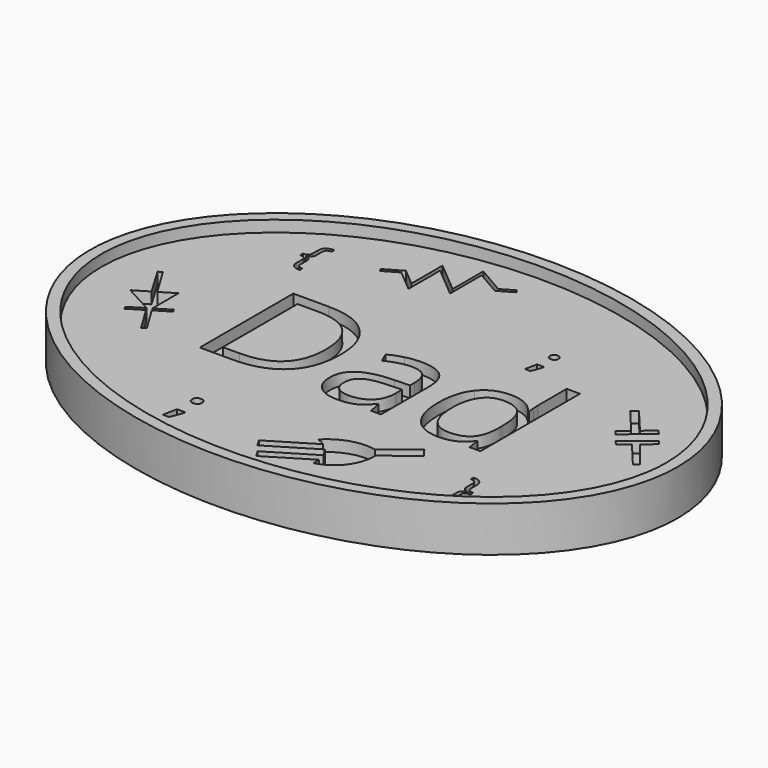
from build123d import *

# Parameters (mm, degrees)
F1_DEPTH       = 10.16
F2_DEPTH       = 7.62
F0_TEXT_SIZE   = 11.1528724018
F3_DEPTH       = 5.08
F4_DEPTH       = 5.08
F0_TEXT_SIZE_2 = 12.9806434011
F5_DEPTH       = 5.08
F6_DEPTH       = 5.08
F0_TEXT_SIZE_3 = 11.0810389742
F7_DEPTH       = 5.08
F0_TEXT_SIZE_4 = 11.3976394965
F8_DEPTH       = 5.08
F0_TEXT_SIZE_5 = 36.8042396278
F9_DEPTH       = 5.08
F10_DEPTH      = 7.62


# Not quite as in the source:
# - Text() gives the source's letters only with a copy of the font that has no kerning and outlines rounded to 1/6400 em; it was checked with that copy


with BuildPart() as f1:
    # F0 (on Top) → F1 (new body)
    with BuildSketch(Plane.XY):
        with BuildLine():
            add(Edge.make_bspline(
                [(-4.4643621796, 33.663463569), (-4.4643621796, 115.0525310167), (-103.5243621796, 74.3579972929), (-202.5843621796, 33.663463569), (-103.5243621796, -7.0310701548), (-4.4643621796, -47.7256038786), (-4.4643621796, 33.663463569)],
                knots=[0, 0, 0, 2.0943951024, 2.0943951024, 4.1887902048, 4.1887902048, 6.2831853072, 6.2831853072, 6.2831853072], degree=2, weights=[1, 0.5, 1, 0.5, 1, 0.5, 1]))
        make_face()
        with BuildLine():
            add(Edge.make_bspline(
                [(-7.0043621796, 33.663463569), (-7.0043621796, 110.6531219655), (-102.2543621796, 72.1582927673), (-197.5043621796, 33.663463569), (-102.2543621796, -4.8313656292), (-7.0043621796, -43.3261948274), (-7.0043621796, 33.663463569)],
                knots=[0, 0, 0, 2.0943951024, 2.0943951024, 4.1887902048, 4.1887902048, 6.2831853072, 6.2831853072, 6.2831853072], degree=2, weights=[1, 0.5, 1, 0.5, 1, 0.5, 1]))
        make_face(mode=Mode.SUBTRACT)
    extrude(amount=F1_DEPTH)

    # F0 (on Top) → F2 (join)
    with BuildSketch(Plane.XY):
        with BuildLine():
            add(Edge.make_bspline(
                [(-7.0043621796, 33.663463569), (-7.0043621796, 110.6531219655), (-102.2543621796, 72.1582927673), (-197.5043621796, 33.663463569), (-102.2543621796, -4.8313656292), (-7.0043621796, -43.3261948274), (-7.0043621796, 33.663463569)],
                knots=[0, 0, 0, 2.0943951024, 2.0943951024, 4.1887902048, 4.1887902048, 6.2831853072, 6.2831853072, 6.2831853072], degree=2, weights=[1, 0.5, 1, 0.5, 1, 0.5, 1]))
        make_face()
        with BuildLine():
            Line((-89.8295319002, -0.3310016424), (-88.0548345603, -0.3310016424))
            Line((-88.0548345603, -0.3310016424), (-87.9615361858, -0.4770338807))
            add(Edge.make_bspline(
                [(-87.9615361858, -0.4770338807), (-88.2901087219, -1.756844191), (-89.0770602281, -3.5132875012)],
                knots=[0, 0, 0, 1, 1, 1], degree=2))
            Line((-89.0770602281, -3.5132875012), (-90.4704511682, -3.5132875012))
            add(Edge.make_bspline(
                [(-90.4704511682, -3.5132875012), (-90.0587213853, -1.8278320846), (-89.8295319002, -0.3310016424)],
                knots=[0, 0, 0, 1, 1, 1], degree=2))
        make_face(mode=Mode.SUBTRACT)
        with BuildLine():
            add(Edge.make_bspline(
                [(-89.8366306896, 3.5033587247), (-90.1276810534, 3.7822397353), (-90.1276810534, 4.3014654713)],
                knots=[0, 0, 0, 1, 1, 1], degree=2))
            add(Edge.make_bspline(
                [(-90.1276810534, 4.3014654713), (-90.1276810534, 4.8348887861), (-89.8427153662, 5.1066710073)],
                knots=[0, 0, 0, 1, 1, 1], degree=2))
            add(Edge.make_bspline(
                [(-89.8427153662, 5.1066710073), (-89.557749679, 5.3784532285), (-89.0121570111, 5.3784532285)],
                knots=[0, 0, 0, 1, 1, 1], degree=2))
            add(Edge.make_bspline(
                [(-89.0121570111, 5.3784532285), (-88.4868465984, 5.3784532285), (-88.198838573, 5.099572218)],
                knots=[0, 0, 0, 1, 1, 1], degree=2))
            add(Edge.make_bspline(
                [(-88.198838573, 5.099572218), (-87.9108305475, 4.8206912074), (-87.9108305475, 4.3014654713)],
                knots=[0, 0, 0, 1, 1, 1], degree=2))
            add(Edge.make_bspline(
                [(-87.9108305475, 4.3014654713), (-87.9108305475, 3.7883244119), (-88.2049232496, 3.506401063)],
                knots=[0, 0, 0, 1, 1, 1], degree=2))
            add(Edge.make_bspline(
                [(-88.2049232496, 3.506401063), (-88.4990159516, 3.2244777142), (-89.0121570111, 3.2244777142)],
                knots=[0, 0, 0, 1, 1, 1], degree=2))
            add(Edge.make_bspline(
                [(-89.0121570111, 3.2244777142), (-89.5455803259, 3.2244777142), (-89.8366306896, 3.5033587247)],
                knots=[0, 0, 0, 1, 1, 1], degree=2))
        make_face(mode=Mode.SUBTRACT)
        Polygon((-118.0367378645, 26.3920886501), (-124.5097741485, 29.8910271376), (-121.2732560065, 31.8154443726), (-125.1676520587, 38.3651069126), (-124.3550517311, 38.8500457286), (-120.3999676678, 32.3346971795), (-117.1634495258, 34.2591144145), (-117.1634495258, 26.891465071), (-113.9092614484, 28.8729695389), (-113.5129605548, 28.2221319234), (-116.7671486322, 26.2406274555), (-113.2141056663, 20.4055308177), (-114.0826090015, 19.878313636), (-117.626974778, 25.7170715611), (-120.889120197, 23.7307217961), (-121.2854210906, 24.3815594116), align=None, mode=Mode.SUBTRACT)
        with BuildLine():
            add(Edge.make_bspline(
                [(-83.7786674321, 43.3568484078), (-80.3829012602, 39.9610822359), (-80.3829012602, 33.8653800475)],
                knots=[0, 0, 0, 1, 1, 1], degree=2))
            add(Edge.make_bspline(
                [(-80.3829012602, 33.8653800475), (-80.3829012602, 27.3613808258), (-83.9138079995, 23.9196093544)],
                knots=[0, 0, 0, 1, 1, 1], degree=2))
            add(Edge.make_bspline(
                [(-83.9138079995, 23.9196093544), (-87.4447147388, 20.4778378829), (-94.0752285343, 20.4778378829)],
                knots=[0, 0, 0, 1, 1, 1], degree=2))
            Line((-94.0752285343, 20.4778378829), (-101.3555671856, 20.4778378829))
            Line((-101.3555671856, 20.4778378829), (-101.3555671856, 46.7526145797))
            Line((-101.3555671856, 46.7526145797), (-93.3046397671, 46.7526145797))
            add(Edge.make_bspline(
                [(-93.3046397671, 46.7526145797), (-87.1744336041, 46.7526145797), (-83.7786674321, 43.3568484078)],
                knots=[0, 0, 0, 1, 1, 1], degree=2))
        make_face(mode=Mode.SUBTRACT)
        with BuildLine():
            ThreePointArc((-51.5886904567, 7.6679179317), (-53.3790541365, 1.9423006734), (-58.3742709473, -1.3797324552))
            ThreePointArc((-58.3742709473, -1.3797324552), (-58.3301274401, -0.5785521341), (-58.3773278194, 0.2224539085))
            Line((-58.3773278194, 0.2224539085), (-67.8649154268, -5.530545453))
            Line((-67.8649154268, -5.530545453), (-68.812615329, -3.9676414299))
            Line((-68.812615329, -3.9676414299), (-58.8528135071, 2.0716950056))
            Line((-58.8528135071, 2.0716950056), (-59.9996521554, 3.9630096857))
            Line((-59.9996521554, 3.9630096857), (-70.2323505411, -2.2418033517))
            Line((-70.2323505411, -2.2418033517), (-71.2327435613, -0.5920002101))
            Line((-71.2327435613, -0.5920002101), (-61.5128771996, 5.3018462857))
            ThreePointArc((-61.5128771996, 5.3018462857), (-62.3952143516, 5.7939746678), (-63.3388458109, 6.1549024491))
            ThreePointArc((-63.3388458109, 6.1549024491), (-58.7003313213, 9.1012736586), (-53.2173938726, 9.4677663726))
            Line((-53.2173938726, 9.4677663726), (-46.348631382, 14.7932060063))
            Line((-46.348631382, 14.7932060063), (-44.8656130503, 12.8804060516))
            Line((-44.8656130503, 12.8804060516), (-51.5886904567, 7.6679179317))
        make_face(mode=Mode.SUBTRACT)
        with BuildLine():
            Line((-30.4221837222, 6.8950638217), (-30.4221837222, 6.9627373062))
            add(Edge.make_bspline(
                [(-30.4221837222, 6.9627373062), (-31.6634578986, 7.1800048091), (-31.6634578986, 8.3767569562)],
                knots=[0, 0, 0, 1, 1, 1], degree=2))
            Line((-31.6634578986, 8.3767569562), (-31.6634578986, 10.0187293962))
            add(Edge.make_bspline(
                [(-31.6634578986, 10.0187293962), (-31.6634578986, 11.0926007425), (-32.9261026491, 11.1246566036)],
                knots=[0, 0, 0, 1, 1, 1], degree=2))
            Line((-32.9261026491, 11.1246566036), (-32.9261026491, 11.8993399131))
            add(Edge.make_bspline(
                [(-32.9261026491, 11.8993399131), (-31.9020959756, 11.8993399131), (-31.3152956296, 11.4149402345)],
                knots=[0, 0, 0, 1, 1, 1], degree=2))
            add(Edge.make_bspline(
                [(-31.3152956296, 11.4149402345), (-30.7284952837, 10.9305405559), (-30.7284952837, 10.079279356)],
                knots=[0, 0, 0, 1, 1, 1], degree=2))
            Line((-30.7284952837, 10.079279356), (-30.7284952837, 8.3767569562))
            add(Edge.make_bspline(
                [(-30.7284952837, 8.3767569562), (-30.7284952837, 7.8371499613), (-30.3999227076, 7.5833743944)],
                knots=[0, 0, 0, 1, 1, 1], degree=2))
            add(Edge.make_bspline(
                [(-30.3999227076, 7.5833743944), (-30.0713501314, 7.3295988275), (-29.3483123759, 7.3189135405)],
                knots=[0, 0, 0, 1, 1, 1], degree=2))
            Line((-29.3483123759, 7.3189135405), (-29.3483123759, 6.5335449439))
            add(Edge.make_bspline(
                [(-29.3483123759, 6.5335449439), (-30.0268281022, 6.5335449439), (-30.3776616929, 6.2860024611)],
                knots=[0, 0, 0, 1, 1, 1], degree=2))
            add(Edge.make_bspline(
                [(-30.3776616929, 6.2860024611), (-30.7284952837, 6.0384599783), (-30.7284952837, 5.4596735976)],
                knots=[0, 0, 0, 1, 1, 1], degree=2))
            Line((-30.7284952837, 5.4596735976), (-30.7284952837, 3.7731791284))
            add(Edge.make_bspline(
                [(-30.7284952837, 3.7731791284), (-30.7284952837, 2.9219179285), (-31.2983772585, 2.4464226557)],
                knots=[0, 0, 0, 1, 1, 1], degree=2))
            add(Edge.make_bspline(
                [(-31.2983772585, 2.4464226557), (-31.8682592333, 1.970927383), (-32.9261026491, 1.9584612148)],
                knots=[0, 0, 0, 1, 1, 1], degree=2))
            Line((-32.9261026491, 1.9584612148), (-32.9261026491, 2.7384871678))
            add(Edge.make_bspline(
                [(-32.9261026491, 2.7384871678), (-32.3081368826, 2.7491724549), (-31.9857973906, 3.0056193435)],
                knots=[0, 0, 0, 1, 1, 1], degree=2))
            add(Edge.make_bspline(
                [(-31.9857973906, 3.0056193435), (-31.6634578986, 3.2620662322), (-31.6634578986, 3.8301673259)],
                knots=[0, 0, 0, 1, 1, 1], degree=2))
            Line((-31.6634578986, 3.8301673259), (-31.6634578986, 5.4828250528))
            add(Edge.make_bspline(
                [(-31.6634578986, 5.4828250528), (-31.6634578986, 6.1168187498), (-31.3571463371, 6.4507339695)],
                knots=[0, 0, 0, 1, 1, 1], degree=2))
            add(Edge.make_bspline(
                [(-31.3571463371, 6.4507339695), (-31.0508347757, 6.7846491891), (-30.4221837222, 6.8950638217)],
                knots=[0, 0, 0, 1, 1, 1], degree=2))
        make_face(mode=Mode.SUBTRACT)
        with BuildLine():
            Line((-60.6466277598, 20.4778378829), (-62.8606327999, 20.4778378829))
            Line((-62.8606327999, 20.4778378829), (-63.4529510314, 23.2841611546))
            Line((-63.4529510314, 23.2841611546), (-63.5967175925, 23.2841611546))
            add(Edge.make_bspline(
                [(-63.5967175925, 23.2841611546), (-65.0688871776, 21.4324478483), (-66.5324307691, 20.7739969987)],
                knots=[0, 0, 0, 1, 1, 1], degree=2))
            add(Edge.make_bspline(
                [(-66.5324307691, 20.7739969987), (-67.9959743605, 20.1155461491), (-70.1927274133, 20.1155461491)],
                knots=[0, 0, 0, 1, 1, 1], degree=2))
            add(Edge.make_bspline(
                [(-70.1927274133, 20.1155461491), (-73.1198145962, 20.1155461491), (-74.7817560419, 21.6279703713)],
                knots=[0, 0, 0, 1, 1, 1], degree=2))
            add(Edge.make_bspline(
                [(-74.7817560419, 21.6279703713), (-76.4436974876, 23.1403945935), (-76.4436974876, 25.9237152154)],
                knots=[0, 0, 0, 1, 1, 1], degree=2))
            add(Edge.make_bspline(
                [(-76.4436974876, 25.9237152154), (-76.4436974876, 31.8871521676), (-66.9033484966, 32.1746852896)],
                knots=[0, 0, 0, 1, 1, 1], degree=2))
            Line((-66.9033484966, 32.1746852896), (-63.5622136178, 32.283947876))
            Line((-63.5622136178, 32.283947876), (-63.5622136178, 33.5088389762))
            add(Edge.make_bspline(
                [(-63.5622136178, 33.5088389762), (-63.5622136178, 35.8263559402), (-64.5570782203, 36.9304831291)],
                knots=[0, 0, 0, 1, 1, 1], degree=2))
            add(Edge.make_bspline(
                [(-64.5570782203, 36.9304831291), (-65.5519428227, 38.0346103179), (-67.7486958755, 38.0346103179)],
                knots=[0, 0, 0, 1, 1, 1], degree=2))
            add(Edge.make_bspline(
                [(-67.7486958755, 38.0346103179), (-70.2099794006, 38.0346103179), (-73.3153371192, 36.5279367581)],
                knots=[0, 0, 0, 1, 1, 1], degree=2))
            Line((-73.3153371192, 36.5279367581), (-74.2354431099, 38.8109497475))
            add(Edge.make_bspline(
                [(-74.2354431099, 38.8109497475), (-72.7805255121, 39.5987905021), (-71.0467007859, 40.0473421725)],
                knots=[0, 0, 0, 1, 1, 1], degree=2))
            add(Edge.make_bspline(
                [(-71.0467007859, 40.0473421725), (-69.3128760597, 40.495893843), (-67.5646746774, 40.495893843)],
                knots=[0, 0, 0, 1, 1, 1], degree=2))
            add(Edge.make_bspline(
                [(-67.5646746774, 40.495893843), (-64.045269263, 40.495893843), (-62.3459485114, 38.93458899)],
                knots=[0, 0, 0, 1, 1, 1], degree=2))
            add(Edge.make_bspline(
                [(-62.3459485114, 38.93458899), (-60.6466277598, 37.3732841371), (-60.6466277598, 33.922886672)],
                knots=[0, 0, 0, 1, 1, 1], degree=2))
            Line((-60.6466277598, 33.922886672), (-60.6466277598, 20.4778378829))
        make_face(mode=Mode.SUBTRACT)
        with BuildLine():
            Line((-107.2986405569, 57.8742015011), (-107.2986405569, 56.2570350028))
            add(Edge.make_bspline(
                [(-107.2986405569, 56.2570350028), (-107.2986405569, 55.701134019), (-106.9797381117, 55.45019439)],
                knots=[0, 0, 0, 1, 1, 1], degree=2))
            add(Edge.make_bspline(
                [(-106.9797381117, 55.45019439), (-106.6608356664, 55.1992547609), (-106.045685048, 55.1887989431)],
                knots=[0, 0, 0, 1, 1, 1], degree=2))
            Line((-106.045685048, 55.1887989431), (-106.045685048, 54.4255242381))
            add(Edge.make_bspline(
                [(-106.045685048, 54.4255242381), (-107.0808110178, 54.4377226923), (-107.6471678195, 54.9003926333)],
                knots=[0, 0, 0, 1, 1, 1], degree=2))
            add(Edge.make_bspline(
                [(-107.6471678195, 54.9003926333), (-108.2135246211, 55.3630625743), (-108.2135246211, 56.2012706408)],
                knots=[0, 0, 0, 1, 1, 1], degree=2))
            Line((-108.2135246211, 56.2012706408), (-108.2135246211, 57.851547229))
            add(Edge.make_bspline(
                [(-108.2135246211, 57.851547229), (-108.2135246211, 58.4179040306), (-108.5559526566, 58.6601304781)],
                knots=[0, 0, 0, 1, 1, 1], degree=2))
            add(Edge.make_bspline(
                [(-108.5559526566, 58.6601304781), (-108.8983806921, 58.9023569256), (-109.5518693093, 58.9023569256)],
                knots=[0, 0, 0, 1, 1, 1], degree=2))
            Line((-109.5518693093, 58.9023569256), (-109.5518693093, 59.6708595395))
            add(Edge.make_bspline(
                [(-109.5518693093, 59.6708595395), (-108.8443589664, 59.6813153574), (-108.5289417937, 59.9322549865)],
                knots=[0, 0, 0, 1, 1, 1], degree=2))
            add(Edge.make_bspline(
                [(-108.5289417937, 59.9322549865), (-108.2135246211, 60.1831946155), (-108.2135246211, 60.7059855093)],
                knots=[0, 0, 0, 1, 1, 1], degree=2))
            Line((-108.2135246211, 60.7059855093), (-108.2135246211, 62.3719458244))
            add(Edge.make_bspline(
                [(-108.2135246211, 62.3719458244), (-108.2135246211, 63.2153817997), (-107.6253848656, 63.6841509679)],
                knots=[0, 0, 0, 1, 1, 1], degree=2))
            add(Edge.make_bspline(
                [(-107.6253848656, 63.6841509679), (-107.03724511, 64.152920136), (-106.045685048, 64.152920136)],
                knots=[0, 0, 0, 1, 1, 1], degree=2))
            Line((-106.045685048, 64.152920136), (-106.045685048, 63.39487334))
            add(Edge.make_bspline(
                [(-106.045685048, 63.39487334), (-107.2986405569, 63.3635058863), (-107.2986405569, 62.3126961897)],
                knots=[0, 0, 0, 1, 1, 1], degree=2))
            Line((-107.2986405569, 62.3126961897), (-107.2986405569, 60.7059855093))
            add(Edge.make_bspline(
                [(-107.2986405569, 60.7059855093), (-107.2986405569, 59.5349339071), (-108.5115154306, 59.322332277)],
                knots=[0, 0, 0, 1, 1, 1], degree=2))
            Line((-108.5115154306, 59.322332277), (-108.5115154306, 59.2561120971))
            add(Edge.make_bspline(
                [(-108.5115154306, 59.2561120971), (-107.2986405569, 59.0452531032), (-107.2986405569, 57.8742015011)],
                knots=[0, 0, 0, 1, 1, 1], degree=2))
        make_face(mode=Mode.SUBTRACT)
        Polygon((-94.8567953229, 62.9562992311), (-95.2377953229, 63.6162105888), (-91.3383192192, 65.8675741669), (-87.5548717972, 62.6928848305), (-87.5548717972, 71.4052021503), (-80.5931436392, 65.5636186206), (-80.5931436392, 74.1896927357), (-74.3551089592, 70.5872267197), (-71.4755007577, 72.24976929), (-71.0842600542, 71.5745979096), (-74.3838168426, 69.6695979096), (-79.8827212213, 72.8452160595), (-79.8827212213, 63.9552160595), (-86.6928563206, 69.6695979096), (-86.6928563206, 60.7795979096), (-91.5572385345, 64.8612992311), align=None, mode=Mode.SUBTRACT)
        with BuildLine():
            Line((-40.7033304115, 20.4778378829), (-41.10012612, 23.1173919437))
            Line((-41.10012612, 23.1173919437), (-41.2611446684, 23.1173919437))
            add(Edge.make_bspline(
                [(-41.2611446684, 23.1173919437), (-43.325632485, 20.1155461491), (-47.4431067934, 20.1155461491)],
                knots=[0, 0, 0, 1, 1, 1], degree=2))
            add(Edge.make_bspline(
                [(-47.4431067934, 20.1155461491), (-51.3075519543, 20.1155461491), (-53.4554243763, 22.7579755411)],
                knots=[0, 0, 0, 1, 1, 1], degree=2))
            add(Edge.make_bspline(
                [(-53.4554243763, 22.7579755411), (-55.6032967983, 25.4004049332), (-55.6032967983, 30.2712160214)],
                knots=[0, 0, 0, 1, 1, 1], degree=2))
            add(Edge.make_bspline(
                [(-55.6032967983, 30.2712160214), (-55.6032967983, 35.1420271096), (-53.4467983826, 37.8390877949)],
                knots=[0, 0, 0, 1, 1, 1], degree=2))
            add(Edge.make_bspline(
                [(-53.4467983826, 37.8390877949), (-51.2902999669, 40.5361484801), (-47.4431067934, 40.5361484801)],
                knots=[0, 0, 0, 1, 1, 1], degree=2))
            add(Edge.make_bspline(
                [(-47.4431067934, 40.5361484801), (-43.4348950714, 40.5361484801), (-41.295648643, 37.6205626221)],
                knots=[0, 0, 0, 1, 1, 1], degree=2))
            Line((-41.295648643, 37.6205626221), (-41.0598714829, 37.6205626221))
            Line((-41.0598714829, 37.6205626221), (-41.1863860566, 39.0409762452))
            Line((-41.1863860566, 39.0409762452), (-41.2611446684, 40.4268858937))
            Line((-41.2611446684, 40.4268858937), (-41.2611446684, 48.4433093376))
            Line((-41.2611446684, 48.4433093376), (-38.2765508611, 48.4433093376))
            Line((-38.2765508611, 48.4433093376), (-38.2765508611, 20.4778378829))
            Line((-38.2765508611, 20.4778378829), (-40.7033304115, 20.4778378829))
        make_face(mode=Mode.SUBTRACT)
        with BuildLine():
            Line((-51.1307175366, 52.4648435821), (-49.6157317393, 52.4648435821))
            Line((-49.6157317393, 52.4648435821), (-49.5360867717, 52.3401818937))
            add(Edge.make_bspline(
                [(-49.5360867717, 52.3401818937), (-49.8165755707, 51.2476607073), (-50.4883635585, 49.7482576211)],
                knots=[0, 0, 0, 1, 1, 1], degree=2))
            Line((-50.4883635585, 49.7482576211), (-51.6778438359, 49.7482576211))
            add(Edge.make_bspline(
                [(-51.6778438359, 49.7482576211), (-51.326367131, 51.1870612754), (-51.1307175366, 52.4648435821)],
                knots=[0, 0, 0, 1, 1, 1], degree=2))
        make_face(mode=Mode.SUBTRACT)
        with BuildLine():
            add(Edge.make_bspline(
                [(-51.1367774798, 55.7380786104), (-51.3852351505, 55.9761478071), (-51.3852351505, 56.4193893661)],
                knots=[0, 0, 0, 1, 1, 1], degree=2))
            add(Edge.make_bspline(
                [(-51.3852351505, 56.4193893661), (-51.3852351505, 56.8747508114), (-51.1419717168, 57.1067600649)],
                knots=[0, 0, 0, 1, 1, 1], degree=2))
            add(Edge.make_bspline(
                [(-51.1419717168, 57.1067600649), (-50.8987082831, 57.3387693184), (-50.4329583637, 57.3387693184)],
                knots=[0, 0, 0, 1, 1, 1], degree=2))
            add(Edge.make_bspline(
                [(-50.4329583637, 57.3387693184), (-49.9845225677, 57.3387693184), (-49.7386620154, 57.1007001217)],
                knots=[0, 0, 0, 1, 1, 1], degree=2))
            add(Edge.make_bspline(
                [(-49.7386620154, 57.1007001217), (-49.4928014632, 56.862630925), (-49.4928014632, 56.4193893661)],
                knots=[0, 0, 0, 1, 1, 1], degree=2))
            add(Edge.make_bspline(
                [(-49.4928014632, 56.4193893661), (-49.4928014632, 55.9813420441), (-49.7438562525, 55.7406757289)],
                knots=[0, 0, 0, 1, 1, 1], degree=2))
            add(Edge.make_bspline(
                [(-49.7438562525, 55.7406757289), (-49.9949110417, 55.5000094137), (-50.4329583637, 55.5000094137)],
                knots=[0, 0, 0, 1, 1, 1], degree=2))
            add(Edge.make_bspline(
                [(-50.4329583637, 55.5000094137), (-50.888319809, 55.5000094137), (-51.1367774798, 55.7380786104)],
                knots=[0, 0, 0, 1, 1, 1], degree=2))
        make_face(mode=Mode.SUBTRACT)
        Polygon((-23.7639061474, 40.2713489151), (-24.5796442032, 41.2447303534), (-22.4383745174, 43.0392120455), (-27.3328028521, 48.879500675), (-26.1506581866, 49.8701918401), (-21.2562298519, 44.0299032106), (-18.7393555737, 46.1391586881), (-17.9236175179, 45.1657772499), align=None, mode=Mode.SUBTRACT)
        Polygon((-21.2712523136, 37.274422138), (-22.1973136067, 38.3825451136), (-16.2467017399, 43.142231911), (-15.4309636841, 42.1688504728), (-18.0022890176, 40.0139625265), (-13.2413589253, 34.061796279), (-14.2147403635, 33.2460582232), (-19.1091686983, 39.0863468527), align=None, mode=Mode.SUBTRACT)
    extrude(amount=F2_DEPTH)

    # F0 (on Top) → F3 (join)
    with BuildSketch(Plane.XY):
        with Locations((-109.8847128451, 56.1908148229)):
            Text('{', F0_TEXT_SIZE, font='Open Sans', text_align=(TextAlign.LEFT, TextAlign.BOTTOM))
    extrude(amount=F3_DEPTH)

    # F0 (on Top) → F4 (join)
    with BuildSketch(Plane.XY):
        with BuildLine():
            ThreePointArc((-58.3773278194, 0.2224539085), (-58.3301274401, -0.5785521341), (-58.3742709473, -1.3797324552))
            ThreePointArc((-58.3742709473, -1.3797324552), (-53.3790541365, 1.9423006734), (-51.5886904567, 7.6679179317))
            ThreePointArc((-51.5886904567, 7.6679179317), (-51.6442188239, 8.3842232893), (-51.7568103969, 9.0938005596))
            ThreePointArc((-51.7568103969, 9.0938005596), (-52.4807591701, 9.3055569321), (-53.2173938726, 9.4677663726))
            ThreePointArc((-53.2173938726, 9.4677663726), (-58.7003313213, 9.1012736586), (-63.3388458109, 6.1549024491))
            ThreePointArc((-63.3388458109, 6.1549024491), (-62.3952143516, 5.7939746678), (-61.5128771996, 5.3018462857))
            ThreePointArc((-61.5128771996, 5.3018462857), (-60.7080429363, 4.6869307879), (-59.9996521554, 3.9630096857))
            ThreePointArc((-59.9996521554, 3.9630096857), (-59.3515824511, 3.0626181822), (-58.8528135071, 2.0716950056))
            ThreePointArc((-58.8528135071, 2.0716950056), (-58.5521623925, 1.1632497316), (-58.3773278194, 0.2224539085))
        make_face()
        with BuildLine():
            ThreePointArc((-51.7568103969, 9.0938005596), (-51.6442188239, 8.3842232893), (-51.5886904567, 7.6679179317))
            Line((-51.5886904567, 7.6679179317), (-44.8656130503, 12.8804060516))
            Line((-44.8656130503, 12.8804060516), (-46.348631382, 14.7932060063))
            Line((-46.348631382, 14.7932060063), (-53.2173938726, 9.4677663726))
            ThreePointArc((-53.2173938726, 9.4677663726), (-52.4807591701, 9.3055569321), (-51.7568103969, 9.0938005596))
        make_face()
        with BuildLine():
            Line((-70.2323505411, -2.2418033517), (-59.9996521554, 3.9630096857))
            ThreePointArc((-59.9996521554, 3.9630096857), (-60.7080429363, 4.6869307879), (-61.5128771996, 5.3018462857))
            Line((-61.5128771996, 5.3018462857), (-71.2327435613, -0.5920002101))
            Line((-71.2327435613, -0.5920002101), (-70.2323505411, -2.2418033517))
        make_face()
        with BuildLine():
            Line((-67.8649154268, -5.530545453), (-58.3773278194, 0.2224539085))
            ThreePointArc((-58.3773278194, 0.2224539085), (-58.5521623925, 1.1632497316), (-58.8528135071, 2.0716950056))
            Line((-58.8528135071, 2.0716950056), (-68.812615329, -3.9676414299))
            Line((-68.812615329, -3.9676414299), (-67.8649154268, -5.530545453))
        make_face()
    extrude(amount=F4_DEPTH)

    # F0 (on Top) → F5 (join)
    with BuildSketch(Plane.XY):
        with Locations((-90.8700115979, -1.8400014378)):
            Text(';', F0_TEXT_SIZE_2, font='Open Sans', font_style=FontStyle.BOLD, text_align=(TextAlign.LEFT, TextAlign.BOTTOM))
    extrude(amount=F5_DEPTH)

    # F0 (on Top) → F6 (join)
    with BuildSketch(Plane.XY):
        Polygon((-125.1676520587, 38.3651069126), (-121.2732560065, 31.8154443726), (-120.8366118371, 32.075070776), (-120.3999676678, 32.3346971795), (-124.3550517311, 38.8500457286), align=None)
        Polygon((-121.2732560065, 31.8154443726), (-124.5097741485, 29.8910271376), (-118.0367378645, 26.3920886501), (-117.1634495258, 26.891465071), (-117.1634495258, 34.2591144145), (-120.3999676678, 32.3346971795), (-120.8366118371, 32.075070776), align=None)
        Polygon((-113.9092614484, 28.8729695389), (-117.1634495258, 26.891465071), (-116.7671486322, 26.2406274555), (-113.5129605548, 28.2221319234), align=None)
        Polygon((-117.1634495258, 26.891465071), (-118.0367378645, 26.3920886501), (-117.2324176348, 25.9573209639), (-117.1634495258, 25.9993162674), align=None)
        Polygon((-117.626974778, 25.7170715611), (-118.0367378645, 26.3920886501), (-121.2854210906, 24.3815594116), (-120.889120197, 23.7307217961), align=None)
        Polygon((-117.1634495258, 25.9200409055), (-117.2324176348, 25.9573209639), (-117.626974778, 25.7170715611), (-114.0826090015, 19.878313636), (-113.2141056663, 20.4055308177), (-116.7671486322, 26.2406274555), (-117.1634495258, 25.9993162674), align=None)
        Polygon((-117.2324176348, 25.9573209639), (-118.0367378645, 26.3920886501), (-117.626974778, 25.7170715611), align=None)
        Polygon((-116.7671486322, 26.2406274555), (-117.1634495258, 26.891465071), (-117.1634495258, 25.9993162674), align=None)
    extrude(amount=F6_DEPTH)

    # F0 (on Top) → F7 (join)
    with BuildSketch(Plane.XY):
        Polygon((-91.3383192192, 65.8675741669), (-95.2377953229, 63.6162105888), (-94.8567953229, 62.9562992311), (-91.5572385345, 64.8612992311), (-86.6928563206, 60.7795979096), (-86.6928563206, 69.6695979096), (-79.8827212213, 63.9552160595), (-79.8827212213, 72.8452160595), (-74.3838168426, 69.6695979096), (-71.0842600542, 71.5745979096), (-71.4755007577, 72.24976929), (-74.3551089592, 70.5872267197), (-80.5931436392, 74.1896927357), (-80.5931436392, 65.5636186206), (-87.5548717972, 71.4052021503), (-87.5548717972, 62.6928848305), align=None)
        with Locations((-52.0189320669, 51.1766728014)):
            Text(';', F0_TEXT_SIZE_3, font='Open Sans', font_style=FontStyle.BOLD, text_align=(TextAlign.LEFT, TextAlign.BOTTOM))
    extrude(amount=F7_DEPTH)

    # F0 (on Top) → F8 (join)
    with BuildSketch(Plane.XY):
        Polygon((-27.3328028521, 48.879500675), (-22.4383745174, 43.0392120455), (-21.2562298519, 44.0299032106), (-26.1506581866, 49.8701918401), align=None)
        Polygon((-22.4383745174, 43.0392120455), (-24.5796442032, 41.2447303534), (-23.7639061474, 40.2713489151), (-17.9236175179, 45.1657772499), (-18.7393555737, 46.1391586881), (-21.2562298519, 44.0299032106), align=None)
        Polygon((-16.2467017399, 43.142231911), (-22.1973136067, 38.3825451136), (-21.2712523136, 37.274422138), (-19.1091686983, 39.0863468527), (-18.0022890176, 40.0139625265), (-15.4309636841, 42.1688504728), align=None)
        Polygon((-18.0022890176, 40.0139625265), (-19.1091686983, 39.0863468527), (-14.2147403635, 33.2460582232), (-13.2413589253, 34.061796279), align=None)
        with Locations((-33.3268009126, 3.7624938414)):
            Text('}', F0_TEXT_SIZE_4, font='Open Sans', text_align=(TextAlign.LEFT, TextAlign.BOTTOM))
    extrude(amount=F8_DEPTH)

    # F0 (on Top) → F9 (join)
    with BuildSketch(Plane.XY):
        with Locations((-104.9669831991, 20.4778378829)):
            Text('Dad', F0_TEXT_SIZE_5, font='Open Sans', text_align=(TextAlign.LEFT, TextAlign.BOTTOM))
    extrude(amount=F9_DEPTH)

    # F0 (on Top) → F10 (join)
    with BuildSketch(Plane.XY):
        with BuildLine():
            add(Edge.make_bspline(
                [(-86.366465531, 25.8058266353), (-83.6147735526, 28.4942613269), (-83.6147735526, 33.7561174612)],
                knots=[0, 0, 0, 1, 1, 1], degree=2))
            add(Edge.make_bspline(
                [(-83.6147735526, 33.7561174612), (-83.6147735526, 38.8972096842), (-86.1939456577, 41.5022597703)],
                knots=[0, 0, 0, 1, 1, 1], degree=2))
            add(Edge.make_bspline(
                [(-86.1939456577, 41.5022597703), (-88.7731177629, 44.1073098565), (-93.8624540239, 44.1073098565)],
                knots=[0, 0, 0, 1, 1, 1], degree=2))
            Line((-93.8624540239, 44.1073098565), (-98.301965429, 44.1073098565))
            Line((-98.301965429, 44.1073098565), (-98.301965429, 23.1173919437))
            Line((-98.301965429, 23.1173919437), (-94.5812868291, 23.1173919437))
            add(Edge.make_bspline(
                [(-94.5812868291, 23.1173919437), (-89.1181575094, 23.1173919437), (-86.366465531, 25.8058266353)],
                knots=[0, 0, 0, 1, 1, 1], degree=2))
        make_face()
        with BuildLine():
            add(Edge.make_bspline(
                [(-72.3377245041, 23.4250523844), (-71.360111889, 22.5825803367), (-69.6004091818, 22.5825803367)],
                knots=[0, 0, 0, 1, 1, 1], degree=2))
            add(Edge.make_bspline(
                [(-69.6004091818, 22.5825803367), (-66.8113378975, 22.5825803367), (-65.2212797323, 24.109381215)],
                knots=[0, 0, 0, 1, 1, 1], degree=2))
            add(Edge.make_bspline(
                [(-65.2212797323, 24.109381215), (-63.6312215671, 25.6361820933), (-63.6312215671, 28.3849987405)],
                knots=[0, 0, 0, 1, 1, 1], degree=2))
            Line((-63.6312215671, 28.3849987405), (-63.6312215671, 30.161953435))
            Line((-63.6312215671, 30.161953435), (-66.6158153745, 30.0411895237))
            add(Edge.make_bspline(
                [(-66.6158153745, 30.0411895237), (-70.175475426, 29.91467495), (-71.7454062726, 28.9341870037)],
                knots=[0, 0, 0, 1, 1, 1], degree=2))
            add(Edge.make_bspline(
                [(-71.7454062726, 28.9341870037), (-73.3153371192, 27.9536990573), (-73.3153371192, 25.8892112407)],
                knots=[0, 0, 0, 1, 1, 1], degree=2))
            add(Edge.make_bspline(
                [(-73.3153371192, 25.8892112407), (-73.3153371192, 24.2675244321), (-72.3377245041, 23.4250523844)],
                knots=[0, 0, 0, 1, 1, 1], degree=2))
        make_face()
        with BuildLine():
            add(Edge.make_bspline(
                [(-51.1264060874, 24.5406808981), (-49.7433717701, 22.6170843113), (-47.0635630722, 22.6170843113)],
                knots=[0, 0, 0, 1, 1, 1], degree=2))
            add(Edge.make_bspline(
                [(-47.0635630722, 22.6170843113), (-44.0099613156, 22.6170843113), (-42.635552992, 24.279025757)],
                knots=[0, 0, 0, 1, 1, 1], degree=2))
            add(Edge.make_bspline(
                [(-42.635552992, 24.279025757), (-41.2611446684, 25.9409672027), (-41.2611446684, 29.6443938152)],
                knots=[0, 0, 0, 1, 1, 1], degree=2))
            Line((-41.2611446684, 29.6443938152), (-41.2611446684, 30.2712160214))
            add(Edge.make_bspline(
                [(-41.2611446684, 30.2712160214), (-41.2611446684, 34.4576982791), (-42.6528049793, 36.2461542985)],
                knots=[0, 0, 0, 1, 1, 1], degree=2))
            add(Edge.make_bspline(
                [(-42.6528049793, 36.2461542985), (-44.0444652902, 38.0346103179), (-47.0980670468, 38.0346103179)],
                knots=[0, 0, 0, 1, 1, 1], degree=2))
            add(Edge.make_bspline(
                [(-47.0980670468, 38.0346103179), (-49.7261197828, 38.0346103179), (-51.1177800937, 35.9960004823)],
                knots=[0, 0, 0, 1, 1, 1], degree=2))
            add(Edge.make_bspline(
                [(-51.1177800937, 35.9960004823), (-52.5094404046, 33.9573906466), (-52.5094404046, 30.2367120467)],
                knots=[0, 0, 0, 1, 1, 1], degree=2))
            add(Edge.make_bspline(
                [(-52.5094404046, 30.2367120467), (-52.5094404046, 26.4642774849), (-51.1264060874, 24.5406808981)],
                knots=[0, 0, 0, 1, 1, 1], degree=2))
        make_face()
    extrude(amount=F10_DEPTH)


solid = f1.part
